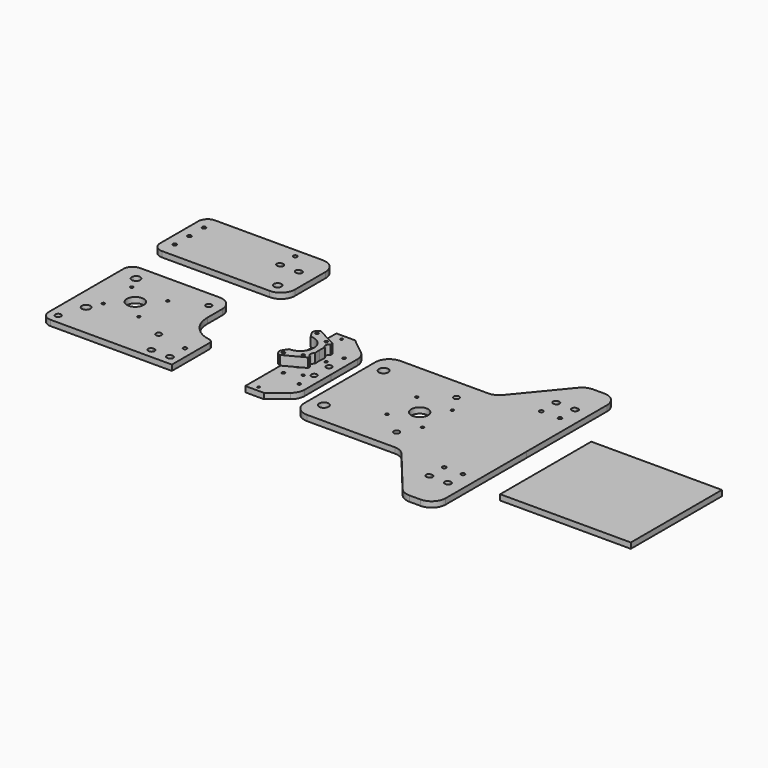
from build123d import *

# Parameters (mm, degrees)
F1_R     = 3
F1_R_2   = 8
F1_R_3   = 1.6000001791
F1_R_4   = 1.2999999784
F1_R_5   = 1.5000003636
F1_R_6   = 1.5863115349
F2_DEPTH = 6
F1_R_7   = 5.0006862955
F1_R_8   = 1.5
F1_R_9   = 2
F1_R_10  = 9
F0_R     = 3.0000000094
F0_R_2   = 4.5
F0_R_3   = 1.5
F0_R_4   = 9
F0_R_5   = 3.0000000194
F0_R_6   = 1.999999576
F0_R_7   = 2
F0_R_8   = 3.9999999458
F0_R_9   = 2.000000225
F3_START = 15
F3_DEPTH = 10


# Not quite as in the source:
# - ends of sketch curves that miss each other by under 0.0002 mm in the source are joined
# - a feature names something its author has since deleted; it is built from what else it names


with BuildPart() as f2:
    # F1 (on Top) → F2 (new body)
    with BuildSketch(Plane.XY):
        with BuildLine():
            ThreePointArc((-70.5460922043, -40.0758998343), (-66.4031669881, -34.8626139586), (-64.9250937577, -28.3697348981))
            Line((-64.9250937577, -28.3697348981), (-64.9250905, 7.000009))
            Line((-64.9250905, 7.000009), (-64.9250937577, 42.3697575026))
            ThreePointArc((-64.9250937577, 42.3697575026), (-66.4031669881, 48.8626365631), (-70.5460922043, 54.0759224388))
            Line((-70.5460922043, 54.0759224388), (-87.925096, 68.0000116045))
            Line((-87.925096, 68.0000116045), (-107.925096, 68.0000116045))
            Line((-107.925096, 68.0000116045), (-107.9250905, 7.0000106045))
            Line((-107.9250905, 7.0000106045), (-107.925096, -53.999989))
            Line((-107.925096, -53.999989), (-87.925096, -53.999989))
            Line((-87.925096, -53.999989), (-70.5460922043, -40.0758998343))
        make_face()
        with BuildLine():
            ThreePointArc((-96.6250960216, -48.499988), (-97.925096, -49.7999879784), (-99.2250959784, -48.499988))
            ThreePointArc((-99.2250959784, -48.499988), (-97.925096, -47.1999880216), (-96.6250960216, -48.499988))
        make_face(mode=Mode.SUBTRACT)
        with BuildLine():
            ThreePointArc((-73.3250933209, -22.9999905), (-73.338781543, -23.2088324214), (-73.379612, -23.414101))
            ThreePointArc((-73.379612, -23.414101), (-75.339204, -24.545472), (-76.470575, -22.58588))
            ThreePointArc((-76.470575, -22.58588), (-74.7162515786, -21.413678543), (-73.3250933209, -22.9999905))
        make_face(mode=Mode.SUBTRACT)
        with Locations((-74.9252350911, -2.9779738972)):
            Circle(F1_R, mode=Mode.SUBTRACT)
        with Locations((-97.9241045, 7.0000113023)):
            Circle(F1_R_2, mode=Mode.SUBTRACT)
        with BuildLine():
            Line((-77.2384336225, 7.0000113023), (-76.8607395663, 0.3841533719))
            ThreePointArc((-76.8607395663, 0.3841533719), (-78.7986049127, -3.2560323112), (-76.4590498384, -6.6520234719))
            Line((-76.4590498384, -6.6520234719), (-76.310734, -9.24999))
            Line((-76.310734, -9.24999), (-97.3903859, -20.3779283069))
            ThreePointArc((-97.3903859, -20.3779283069), (-97.5160428855, -20.4183867764), (-97.6479624833, -20.4135097433))
            ThreePointArc((-97.6479624833, -20.4135097433), (-98.5909482701, -20.1483637824), (-99.4931968154, -19.7669556844))
            ThreePointArc((-99.4931968154, -19.7669556844), (-102.078916495, -16.6287014072), (-101.4778848133, -12.6070913954))
            Line((-101.4778848133, -12.6070913954), (-98.233116289, -7.5124757052))
            ThreePointArc((-98.233116289, -7.5124757052), (-87.76974038, -3.3728695294), (-83.408327999, 7.0000113023))
            ThreePointArc((-83.408327999, 7.0000113023), (-87.76974038, 17.3728921339), (-98.233116289, 21.5124983097))
            Line((-98.233116289, 21.5124983097), (-101.4778848133, 26.607114))
            ThreePointArc((-101.4778848133, 26.607114), (-102.078916495, 30.6287240118), (-99.4931968154, 33.766978289))
            ThreePointArc((-99.4931968154, 33.766978289), (-98.5909482701, 34.1483863869), (-97.6479624833, 34.4135323478))
            ThreePointArc((-97.6479624833, 34.4135323478), (-97.5160428855, 34.418409381), (-97.3903859, 34.3779509114))
            Line((-97.3903859, 34.3779509114), (-76.310734, 23.2500126045))
            Line((-76.310734, 23.2500126045), (-76.4590498384, 20.6520460764))
            ThreePointArc((-76.4590498384, 20.6520460764), (-78.7986049127, 17.2560549158), (-76.8607395663, 13.6158692326))
            Line((-76.8607395663, 13.6158692326), (-77.2384336225, 7.0000113023))
        make_face(mode=Mode.SUBTRACT)
        with Locations((-74.9252350911, 16.9779965017)):
            Circle(F1_R, mode=Mode.SUBTRACT)
        with Locations((-74.9250935, 37.0000131045)):
            Circle(F1_R_3, mode=Mode.SUBTRACT)
        with Locations((-97.925096, 62.5000106045)):
            Circle(F1_R_4, mode=Mode.SUBTRACT)
        with BuildLine():
            ThreePointArc((-76.4590498384, -6.6520234719), (-78.7986049127, -3.2560323112), (-76.8607395663, 0.3841533719))
            Line((-76.8607395663, 0.3841533719), (-77.2384336225, 7.0000113023))
            Line((-77.2384336225, 7.0000113023), (-76.8607395663, 13.6158692326))
            ThreePointArc((-76.8607395663, 13.6158692326), (-78.7986049127, 17.2560549158), (-76.4590498384, 20.6520460764))
            Line((-76.4590498384, 20.6520460764), (-76.310734, 23.2500126045))
            Line((-76.310734, 23.2500126045), (-97.3903859, 34.3779509114))
            ThreePointArc((-97.3903859, 34.3779509114), (-97.5160428855, 34.418409381), (-97.6479624833, 34.4135323478))
            ThreePointArc((-97.6479624833, 34.4135323478), (-98.5909482701, 34.1483863869), (-99.4931968154, 33.766978289))
            ThreePointArc((-99.4931968154, 33.766978289), (-102.078916495, 30.6287240118), (-101.4778848133, 26.607114))
            Line((-101.4778848133, 26.607114), (-98.233116289, 21.5124983097))
            ThreePointArc((-98.233116289, 21.5124983097), (-87.76974038, 17.3728921339), (-83.408327999, 7.0000113023))
            ThreePointArc((-83.408327999, 7.0000113023), (-87.76974038, -3.3728695294), (-98.233116289, -7.5124757052))
            Line((-98.233116289, -7.5124757052), (-101.4778848133, -12.6070913954))
            ThreePointArc((-101.4778848133, -12.6070913954), (-102.078916495, -16.6287014072), (-99.4931968154, -19.7669556844))
            ThreePointArc((-99.4931968154, -19.7669556844), (-98.5909482701, -20.1483637824), (-97.6479624833, -20.4135097433))
            ThreePointArc((-97.6479624833, -20.4135097433), (-97.5160428855, -20.4183867764), (-97.3903859, -20.3779283069))
            Line((-97.3903859, -20.3779283069), (-76.310734, -9.24999))
            Line((-76.310734, -9.24999), (-76.4590498384, -6.6520234719))
        make_face()
        with BuildLine():
            ThreePointArc((-96.3387814651, -15.499988), (-97.925093, -17.0862995349), (-99.5114045349, -15.499988))
            ThreePointArc((-99.5114045349, -15.499988), (-97.925093, -13.9136764651), (-96.3387814651, -15.499988))
        make_face(mode=Mode.SUBTRACT)
        with BuildLine():
            ThreePointArc((-80.9241056364, -8.49999), (-82.424106, -9.9999903636), (-83.9241063636, -8.49999))
            ThreePointArc((-83.9241063636, -8.49999), (-82.424106, -6.9999896364), (-80.9241056364, -8.49999))
        make_face(mode=Mode.SUBTRACT)
        with Locations((-82.424106, 22.5000126045)):
            Circle(F1_R_5, mode=Mode.SUBTRACT)
        with Locations((-97.925093, 29.5000106045)):
            Circle(F1_R_6, mode=Mode.SUBTRACT)
    extrude(amount=F2_DEPTH)


with BuildPart() as f2b:
    # F1 (on Top) → F2, piece 2 (new body)
    with BuildSketch(Plane.XY):
        with BuildLine():
            Line((150.0511015414, -108.0441608115), (150.0748155087, -0.0220752018))
            Line((150.0748155087, -0.0220752018), (150.0748155087, 108.0000130108))
            ThreePointArc((150.0748155087, 108.0000130108), (145.6814172265, 118.6066147286), (135.0748155087, 123.0000130108))
            Line((135.0748155087, 123.0000130108), (123.1405434494, 123.0000130108))
            ThreePointArc((123.1405434494, 123.0000130108), (116.7449964508, 121.5682471844), (111.5703728701, 117.5462768227))
            Line((111.5703728701, 117.5462768227), (70.6629846202, 67.9660987204))
            ThreePointArc((70.6629846202, 67.9660987204), (65.4883610395, 63.9441283587), (59.0928140409, 62.5123625322))
            Line((59.0928140409, 62.5123625322), (-34.9077528063, 62.5123625322))
            ThreePointArc((-34.9077528063, 62.5123625322), (-45.5137723943, 58.1195463479), (-49.9077527159, 47.5140089988))
            Line((-49.9077527159, 47.5140089988), (-49.912968078, -0.0001236552))
            Line((-49.912968078, -0.0001236552), (-49.9181834401, -47.5142563092))
            ThreePointArc((-49.9181834401, -47.5142563092), (-45.526531446, -58.1207580083), (-34.9214764635, -62.5159024143))
            Line((-34.9214764635, -62.5159024143), (59.0790881186, -62.5365382528))
            ThreePointArc((59.0790881186, -62.5365382528), (65.4743206491, -63.9697080519), (70.6480611665, -67.992814296))
            Line((70.6480611665, -67.992814296), (111.5445641501, -117.5819715565))
            ThreePointArc((111.5445641501, -117.5819715565), (116.7183046675, -121.6050778005), (123.113537198, -123.0382475997))
            Line((123.113537198, -123.0382475997), (135.0478089698, -123.040867517))
            ThreePointArc((135.0478089698, -123.040867517), (145.6553749098, -118.649797796), (150.0511015414, -108.0441608115))
        make_face()
        with Locations((-34.91611, -39.987817)):
            Circle(F1_R_7, mode=Mode.SUBTRACT)
        with Locations((43.0849139086, -40.0816046936)):
            Circle(F1_R, mode=Mode.SUBTRACT)
        with Locations((16.728823, -19.9904944748)):
            Circle(F1_R_8, mode=Mode.SUBTRACT)
        with Locations((54.728823, -19.9904944748)):
            Circle(F1_R_8, mode=Mode.SUBTRACT)
        with BuildLine():
            Line((113.574883364, -82.021298), (114.074883364, -82.021298))
            Line((114.074883364, -82.021298), (114.574883364, -82.021298))
            ThreePointArc((114.574883364, -82.021298), (117.574883364, -85.021298), (114.574883364, -88.021298))
            Line((114.574883364, -88.021298), (114.074883364, -88.021298))
            Line((114.074883364, -88.021298), (113.574883364, -88.021298))
            ThreePointArc((113.574883364, -88.021298), (110.574883364, -85.021298), (113.574883364, -82.021298))
        make_face(mode=Mode.SUBTRACT)
        with BuildLine():
            Line((133.574883364, -82.021298), (134.574883364, -82.021298))
            ThreePointArc((134.574883364, -82.021298), (137.574883364, -85.021298), (134.574883364, -88.021298))
            Line((134.574883364, -88.021298), (133.574883364, -88.021298))
            ThreePointArc((133.574883364, -88.021298), (130.574883364, -85.021298), (133.574883364, -82.021298))
        make_face(mode=Mode.SUBTRACT)
        with Locations((114.074883364, -65.021298)):
            Circle(F1_R_9, mode=Mode.SUBTRACT)
        with Locations((134.074883364, -65.021298)):
            Circle(F1_R_9, mode=Mode.SUBTRACT)
        with Locations((-34.9073319081, 39.9842764827)):
            Circle(F1_R_7, mode=Mode.SUBTRACT)
        with Locations((35.728823, 0)):
            Circle(F1_R_10, mode=Mode.SUBTRACT)
        with Locations((16.728823, 19.9904944748)):
            Circle(F1_R_8, mode=Mode.SUBTRACT)
        with Locations((54.728823, 19.9904944748)):
            Circle(F1_R_8, mode=Mode.SUBTRACT)
        with Locations((43.09371071, 40.0609406971)):
            Circle(F1_R, mode=Mode.SUBTRACT)
        with Locations((114.0891534376, 64.9850490546)):
            Circle(F1_R_9, mode=Mode.SUBTRACT)
        with Locations((134.0891529557, 64.9806584771)):
            Circle(F1_R_9, mode=Mode.SUBTRACT)
        with BuildLine():
            ThreePointArc((114.5942025896, 87.9849387359), (117.5935439307, 84.9842802216), (114.5928854164, 81.9849388805))
            Line((114.5928854164, 81.9849388805), (114.0928852983, 81.985048645))
            Line((114.0928852983, 81.985048645), (113.5928854405, 81.9851584094))
            ThreePointArc((113.5928854405, 81.9851584094), (110.5935440994, 84.9858169237), (113.5942026137, 87.9851582648))
            Line((113.5942026137, 87.9851582648), (114.0942027318, 87.9850485004))
            Line((114.0942027318, 87.9850485004), (114.5942025896, 87.9849387359))
        make_face(mode=Mode.SUBTRACT)
        with BuildLine():
            ThreePointArc((133.5928849586, 81.9807678319), (130.5935436175, 84.9814263463), (133.5942021318, 87.9807676874))
            Line((133.5942021318, 87.9807676874), (134.5942021077, 87.9805481585))
            ThreePointArc((134.5942021077, 87.9805481585), (137.5935434488, 84.9798896442), (134.5928849345, 81.9805483031))
            Line((134.5928849345, 81.9805483031), (133.5928849586, 81.9807678319))
        make_face(mode=Mode.SUBTRACT)
    extrude(amount=F2_DEPTH)


with BuildPart() as f2c:
    # F1 (on Top) → F2, piece 3 (new body)
    with BuildSketch(Plane.XY):
        Polygon((321.101666, 48.0782673955), (194.101666, 48.0782673955), (181.101666, 48.0782673955), (181.101666, -73.9217326045), (321.101666, -73.9217326045), align=None)
    extrude(amount=F2_DEPTH)


with BuildPart() as f2d:
    # F0 (on Top) → F2, piece 4 (new body)
    with BuildSketch(Plane.XY):
        with BuildLine():
            Line((-220.088257, -62.11128), (-180.088257, -62.11128))
            Line((-180.088257, -62.11128), (-180.088257, -42.11128))
            Line((-180.088257, -42.11128), (-180.088257, -11.7581270741))
            ThreePointArc((-180.088257, -11.7581270741), (-181.2790880743, -8.519264296), (-184.2843498382, -6.8231768945))
            Line((-184.2843498382, -6.8231768945), (-184.911699971, -6.7209810776))
            ThreePointArc((-184.911699971, -6.7209810776), (-202.9432705542, 3.4555433313), (-210.088257, 22.88872))
            Line((-210.088257, 22.88872), (-210.088257, 42.88872))
            ThreePointArc((-210.088257, 42.88872), (-214.4816552822, 53.4953217178), (-225.088257, 57.88872))
            Line((-225.088257, 57.88872), (-310.088257, 57.88872))
            ThreePointArc((-310.088257, 57.88872), (-317.1593248119, 54.9597878119), (-320.088257, 47.88872))
            Line((-320.088257, 47.88872), (-320.088257, -52.11128))
            ThreePointArc((-320.088257, -52.11128), (-317.1593248119, -59.1823478119), (-310.088257, -62.11128))
            Line((-310.088257, -62.11128), (-220.088257, -62.11128))
        make_face()
        with Locations((-310.0601935, -51.8858805)):
            Circle(F0_R, mode=Mode.SUBTRACT)
        with Locations((-301.0329645, -25.9005545)):
            Circle(F0_R_2, mode=Mode.SUBTRACT)
        with Locations((-293.940429, -11.510976)):
            Circle(F0_R_3, mode=Mode.SUBTRACT)
        with Locations((-255.940429, -11.510976)):
            Circle(F0_R_3, mode=Mode.SUBTRACT)
        with Locations((-293.940429, 26.489024)):
            Circle(F0_R_3, mode=Mode.SUBTRACT)
        with Locations((-300.9256081469, 40.9622196337)):
            Circle(F0_R_2, mode=Mode.SUBTRACT)
        with Locations((-274.940429, 7.489024)):
            Circle(F0_R_4, mode=Mode.SUBTRACT)
        with Locations((-254.7548115253, 25.8758086711)):
            Circle(F0_R_3, mode=Mode.SUBTRACT)
        with Locations((-223.005992, -26.025945)):
            Circle(F0_R_5, mode=Mode.SUBTRACT)
        with BuildLine():
            Line((-210.588242, -49.094027), (-210.088242, -49.094027))
            Line((-210.088242, -49.094027), (-209.588242, -49.094027))
            ThreePointArc((-209.588242, -49.094027), (-206.588242, -52.094027), (-209.588242, -55.094027))
            Line((-209.588242, -55.094027), (-210.088242, -55.094027))
            Line((-210.088242, -55.094027), (-210.588242, -55.094027))
            ThreePointArc((-210.588242, -55.094027), (-213.588242, -52.094027), (-210.588242, -49.094027))
        make_face(mode=Mode.SUBTRACT)
        with BuildLine():
            ThreePointArc((-189.6345736902, -55.094027), (-190.088272, -55.1285324643), (-190.5419703098, -55.094027))
            Line((-190.5419703098, -55.094027), (-190.588272, -55.094027))
            ThreePointArc((-190.588272, -55.094027), (-193.588272, -52.094027), (-190.588272, -49.094027))
            Line((-190.588272, -49.094027), (-189.588272, -49.094027))
            ThreePointArc((-189.588272, -49.094027), (-186.588272, -52.094027), (-189.588272, -55.094027))
            Line((-189.588272, -55.094027), (-189.6345736902, -55.094027))
        make_face(mode=Mode.SUBTRACT)
        with Locations((-190.072526, -32.094066)):
            Circle(F0_R_6, mode=Mode.SUBTRACT)
        with Locations((-222.898635298, 40.8370464579)):
            Circle(F0_R_5, mode=Mode.SUBTRACT)
        with BuildLine():
            ThreePointArc((-210.088242, -49.0940270348), (-209.8373632191, -49.1045354666), (-209.588242, -49.1359871438))
            Line((-209.588242, -49.1359871438), (-209.588242, -49.094027))
            Line((-209.588242, -49.094027), (-210.088242, -49.094027))
        make_face()
        with BuildLine():
            Line((-209.588242, -55.094027), (-209.588242, -55.0520668562))
            ThreePointArc((-209.588242, -55.0520668562), (-209.8373632191, -55.0835185334), (-210.088242, -55.0940269652))
            Line((-210.088242, -55.094027), (-209.588242, -55.094027))
        make_face()
        with BuildLine():
            ThreePointArc((-210.588242, -49.1359871438), (-210.3391207809, -49.1045354666), (-210.088242, -49.0940270348))
            Line((-210.088242, -49.094027), (-210.588242, -49.094027))
            Line((-210.588242, -49.094027), (-210.588242, -49.1359871438))
        make_face()
        with BuildLine():
            Line((-210.588242, -55.094027), (-210.088242, -55.094027))
            ThreePointArc((-210.088242, -55.0940269652), (-210.3391207809, -55.0835185334), (-210.588242, -55.0520668562))
            Line((-210.588242, -55.0520668562), (-210.588242, -55.094027))
        make_face()
    extrude(amount=F2_DEPTH)


with BuildPart() as f2e:
    # F0 (on Top) → F2, piece 5 (new body)
    with BuildSketch(Plane.XY):
        with BuildLine():
            Line((-315.1174431717, 93.320559795), (-199.6354959271, 93.320559795))
            ThreePointArc((-199.6354959271, 93.320559795), (-189.0288942093, 97.7139580772), (-184.6354959271, 108.320559795))
            Line((-184.6354959271, 108.320559795), (-184.6354959271, 149.5247143484))
            ThreePointArc((-184.6354959271, 149.5247143484), (-189.0288942093, 160.1313160662), (-199.6354959271, 164.5247143484))
            Line((-199.6354959271, 164.5247143484), (-315.1174431717, 164.5247143484))
            ThreePointArc((-315.1174431717, 164.5247143484), (-322.1885109836, 161.5957821602), (-325.1174431717, 154.5247143484))
            Line((-325.1174431717, 154.5247143484), (-325.1174431717, 103.320559795))
            ThreePointArc((-325.1174431717, 103.320559795), (-322.1885109836, 96.2494919831), (-315.1174431717, 93.320559795))
        make_face()
        with Locations((-314.1155334271, 109.3954220414)):
            Circle(F0_R_7, mode=Mode.SUBTRACT)
        with Locations((-314.1155334271, 128.9226370717)):
            Circle(F0_R_7, mode=Mode.SUBTRACT)
        with Locations((-314.1155334271, 148.4498521019)):
            Circle(F0_R_7, mode=Mode.SUBTRACT)
        with Locations((-200.7297894271, 105.459195295)):
            Circle(F0_R_8, mode=Mode.SUBTRACT)
        with BuildLine():
            Line((-222.7727389271, 138.645285795), (-221.7727389271, 138.645285795))
            ThreePointArc((-221.7727389271, 138.645285795), (-218.7727389271, 135.645285795), (-221.7727389271, 132.645285795))
            Line((-221.7727389271, 132.645285795), (-222.7727389271, 132.645285795))
            ThreePointArc((-222.7727389271, 132.645285795), (-225.7727389271, 135.645285795), (-222.7727389271, 138.645285795))
        make_face(mode=Mode.SUBTRACT)
        with Locations((-222.1017524271, 155.645285795)):
            Circle(F0_R_9, mode=Mode.SUBTRACT)
        with BuildLine():
            Line((-201.7727503585, 132.645285795), (-202.7727503585, 132.645285795))
            ThreePointArc((-202.7727503585, 132.645285795), (-205.7727503585, 135.645285795), (-202.7727503585, 138.645285795))
            Line((-202.7727503585, 138.645285795), (-201.7727503585, 138.645285795))
            ThreePointArc((-201.7727503585, 138.645285795), (-198.7727503585, 135.645285795), (-201.7727503585, 132.645285795))
        make_face(mode=Mode.SUBTRACT)
    extrude(amount=F2_DEPTH)


with BuildPart() as f3:
    # F1 (on Top) → F3 (new body)
    with BuildSketch(Plane.XY.offset(F3_START)):
        with BuildLine():
            ThreePointArc((-76.4590498384, -6.6520234719), (-78.7986049127, -3.2560323112), (-76.8607395663, 0.3841533719))
            Line((-76.8607395663, 0.3841533719), (-77.2384336225, 7.0000113023))
            Line((-77.2384336225, 7.0000113023), (-76.8607395663, 13.6158692326))
            ThreePointArc((-76.8607395663, 13.6158692326), (-78.7986049127, 17.2560549158), (-76.4590498384, 20.6520460764))
            Line((-76.4590498384, 20.6520460764), (-76.310734, 23.2500126045))
            Line((-76.310734, 23.2500126045), (-97.3903859, 34.3779509114))
            ThreePointArc((-97.3903859, 34.3779509114), (-97.5160428855, 34.418409381), (-97.6479624833, 34.4135323478))
            ThreePointArc((-97.6479624833, 34.4135323478), (-98.5909482701, 34.1483863869), (-99.4931968154, 33.766978289))
            ThreePointArc((-99.4931968154, 33.766978289), (-102.078916495, 30.6287240118), (-101.4778848133, 26.607114))
            Line((-101.4778848133, 26.607114), (-98.233116289, 21.5124983097))
            ThreePointArc((-98.233116289, 21.5124983097), (-87.76974038, 17.3728921339), (-83.408327999, 7.0000113023))
            ThreePointArc((-83.408327999, 7.0000113023), (-87.76974038, -3.3728695294), (-98.233116289, -7.5124757052))
            Line((-98.233116289, -7.5124757052), (-101.4778848133, -12.6070913954))
            ThreePointArc((-101.4778848133, -12.6070913954), (-102.078916495, -16.6287014072), (-99.4931968154, -19.7669556844))
            ThreePointArc((-99.4931968154, -19.7669556844), (-98.5909482701, -20.1483637824), (-97.6479624833, -20.4135097433))
            ThreePointArc((-97.6479624833, -20.4135097433), (-97.5160428855, -20.4183867764), (-97.3903859, -20.3779283069))
            Line((-97.3903859, -20.3779283069), (-76.310734, -9.24999))
            Line((-76.310734, -9.24999), (-76.4590498384, -6.6520234719))
        make_face()
        with BuildLine():
            ThreePointArc((-96.3387814651, -15.499988), (-97.925093, -17.0862995349), (-99.5114045349, -15.499988))
            ThreePointArc((-99.5114045349, -15.499988), (-97.925093, -13.9136764651), (-96.3387814651, -15.499988))
        make_face(mode=Mode.SUBTRACT)
        with BuildLine():
            ThreePointArc((-80.9241056364, -8.49999), (-82.424106, -9.9999903636), (-83.9241063636, -8.49999))
            ThreePointArc((-83.9241063636, -8.49999), (-82.424106, -6.9999896364), (-80.9241056364, -8.49999))
        make_face(mode=Mode.SUBTRACT)
        with Locations((-82.424106, 22.5000126045)):
            Circle(F1_R_5, mode=Mode.SUBTRACT)
        with Locations((-97.925093, 29.5000106045)):
            Circle(F1_R_6, mode=Mode.SUBTRACT)
    extrude(amount=F3_DEPTH)


solid = Compound([f2.part, f2b.part, f2c.part, f2d.part, f2e.part, f3.part])
